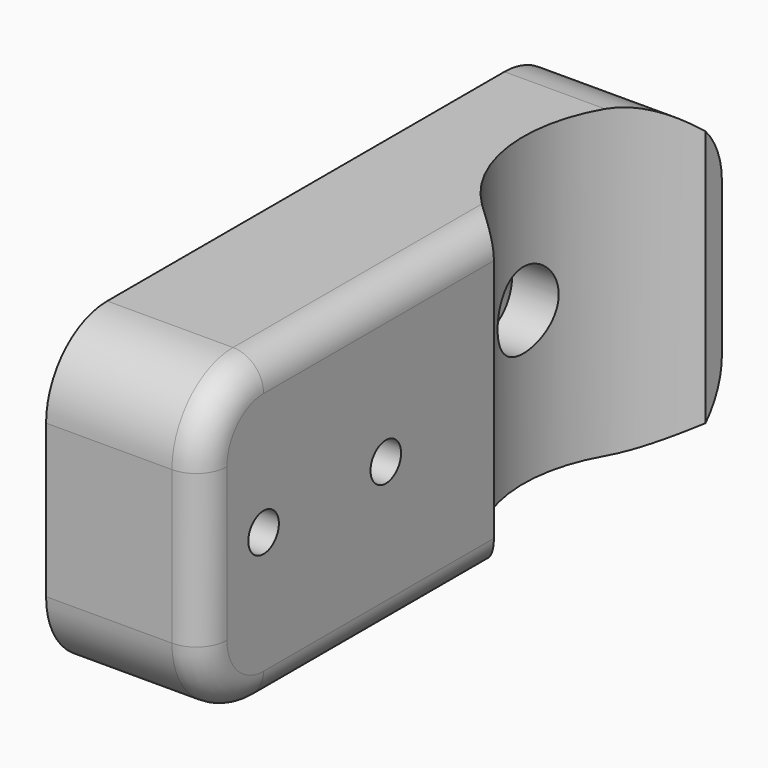
from build123d import *

# Parameters (mm, degrees)
F0_R        = 1.5875
F0_R_2      = 3.175
F1_DEPTH    = 13
F3_DEPTH    = 37.5
F4_T1_DEPTH = 44.75
F5_R        = 2.54
F6_SIZE     = 3.175


# Not quite as in the source:
# - a fillet or chamfer that OpenCascade refuses, or shapes differently, is made with other operations: its cross-section is extruded or revolved along the edge and cut away or added
# - a feature names something its author has since deleted; it is built from what else it names


with BuildPart() as f1:
    # F0 (on Right) → F1 (new body)
    with BuildSketch(Plane.YZ):
        Polygon((0, 0), (0, -12.7), (53.975, -12.7), (53.975, 12.7), (0, 12.7), align=None)
        with Locations((6.35, 0)):
            Circle(F0_R, mode=Mode.SUBTRACT)
        with Locations((19.05, 0)):
            Circle(F0_R, mode=Mode.SUBTRACT)
        with Locations((41.275, 0)):
            Circle(F0_R_2, mode=Mode.SUBTRACT)
    extrude(amount=-F1_DEPTH)

    # F2 (on Top) → F3 (cut, symmetric)
    with BuildSketch(Plane.XY):
        with BuildLine():
            Line((0, 30.2764773719), (0, 52.2735226281))
            ThreePointArc((0, 52.2735226281), (-6.35, 41.275), (0, 30.2764773719))
        make_face()
    extrude(amount=F3_DEPTH, both=True, mode=Mode.SUBTRACT)

    # F4: fillet of radius 6.35 on 4 edges, made by hand

    # F4_s2 → F4_t1 (cut)
    with BuildSketch(Plane.YZ.offset(-28.875)):
        with BuildLine():
            ThreePointArc((0, -6.35), (1.8598719395, -10.8401280605), (6.35, -12.7))
            Line((6.35, -12.7), (0, -12.7))
            Line((0, -12.7), (0, -6.35))
        make_face()
        with BuildLine():
            ThreePointArc((0, 6.35), (1.8598719395, 10.8401280605), (6.35, 12.7))
            Line((6.35, 12.7), (0, 12.7))
            Line((0, 12.7), (0, 6.35))
        make_face()
        with BuildLine():
            ThreePointArc((47.625, -12.7), (52.1151280605, -10.8401280605), (53.975, -6.35))
            Line((53.975, -6.35), (53.975, -12.7))
            Line((53.975, -12.7), (47.625, -12.7))
        make_face()
        with BuildLine():
            ThreePointArc((47.625, 12.7), (52.1151280605, 10.8401280605), (53.975, 6.35))
            Line((53.975, 6.35), (53.975, 12.7))
            Line((53.975, 12.7), (47.625, 12.7))
        make_face()
    extrude(amount=F4_T1_DEPTH, mode=Mode.SUBTRACT)

    # F5
    f5_edges = [f1.edges().sort_by_distance(p)[0] for p in [
        (-6.5, 0, 6.35),
        (0, 0, 0),
        (0, 1.859872, -10.840128),
        (0, 1.859872, 10.840128),
        (0, 18.313239, 12.7),
        (0, 18.313239, -12.7),
    ]]
    fillet(f5_edges, radius=F5_R)

    # F6
    f6_edges = [f1.edges().sort_by_distance(p)[0] for p in [
        (-13, 38.1, 0),
    ]]
    chamfer(f6_edges, length=F6_SIZE)


solid = f1.part
